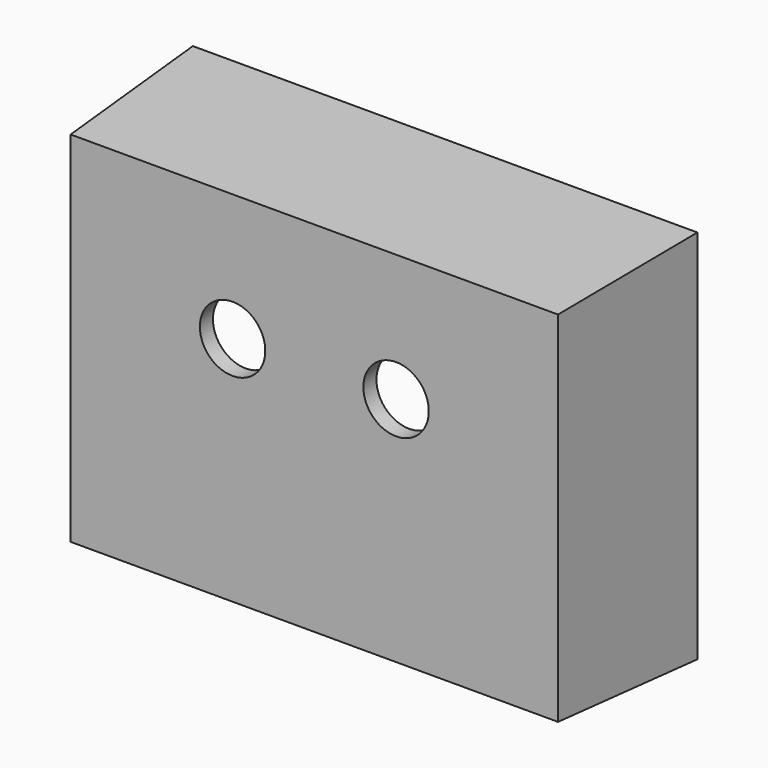
from build123d import *

# Parameters (mm, degrees)
F0_W     = 75.7237523794
F0_H     = 55.7212531567
F1_DEPTH = 25.4
F1_TAPER = -3
F2_T     = -2.54
F3_R     = 5.08
F4_DEPTH = 2.5410001


# Not quite as in the source:
# - a feature of the source that left no trace in its solid (it failed there, or was rolled back) is left out


with BuildPart() as f1:
    # F0 (on Front) → F1 (new body)
    with BuildSketch(Plane.XZ):
        Rectangle(F0_W, F0_H)
    extrude(amount=-F1_DEPTH, taper=F1_TAPER)

    # F2
    f2_openings = [f1.faces().sort_by_distance(p)[0] for p in [
        (0, 25.4, 0),
    ]]
    offset(amount=F2_T, openings=f2_openings)

    # F3 (on face) → F4 (cut, through all)
    with BuildSketch(Plane(origin=(0, 2.54, 0), x_dir=(-1, 0, 0), z_dir=(0, 1, 0))):
        with Locations((12.7, 8.0962497741)):
            Circle(F3_R)
        with Locations((-12.7, 8.0962497741)):
            Circle(F3_R)
    extrude(amount=-F4_DEPTH, mode=Mode.SUBTRACT)


solid = f1.part
